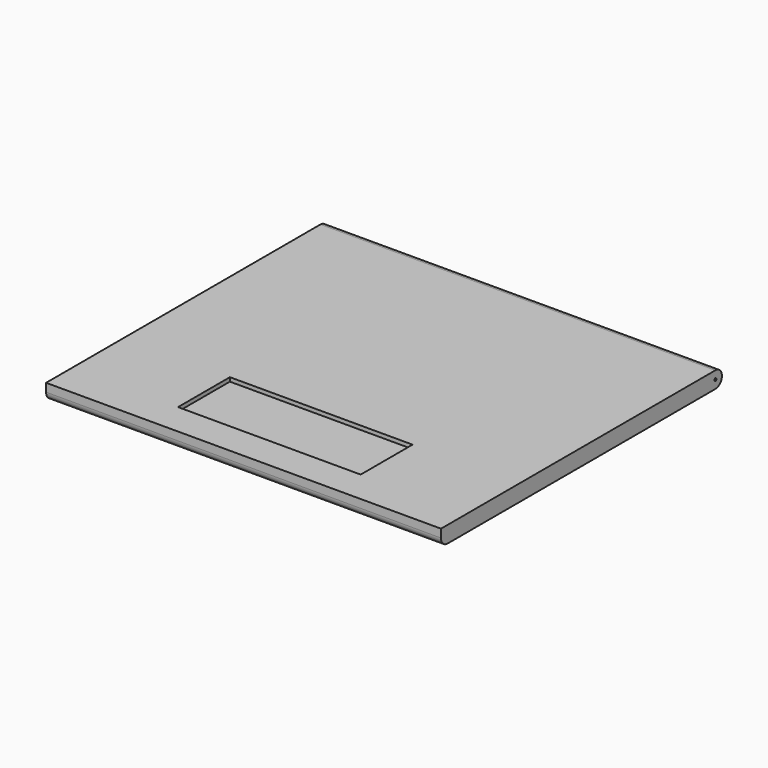
from build123d import *

# Parameters (mm, degrees)
F2_DEPTH = 5
F3_DEPTH = 1.2
F4_R     = 0.4
F5_DEPTH = 2.5
F6_R     = 0.4
F7_DEPTH = 5
F8_R     = 2.49999
F9_R     = 2.5


# Not quite as in the source:
# - a fillet or chamfer is up to 0.001 mm smaller than in the source, because OpenCascade refuses the exact size


with BuildPart() as f2:
    # F1 (on Top) → F2 (new body)
    with BuildSketch(Plane.XY):
        Polygon((-60, -46.1892857143), (-0.7, -46.1892857143), (60, -46.1892857143), (60, 60.5107142857), (0, 60.5107142857), (-60, 60.5107142857), align=None)
        Polygon((-27.75, -16.6892857143), (0, -16.6892857143), (27.75, -16.6892857143), (27.75, -36.3892857143), (-0.7, -36.3892857143), (-27.75, -36.3892857143), align=None, mode=Mode.SUBTRACT)
        Polygon((27.75, -16.6892857143), (0, -16.6892857143), (-27.75, -16.6892857143), (-27.75, -36.3892857143), (-0.7, -36.3892857143), (27.75, -36.3892857143), align=None)
    extrude(amount=-F2_DEPTH)

    # F1 (on Top) → F3 (cut)
    with BuildSketch(Plane.XY):
        Polygon((27.75, -16.6892857143), (0, -16.6892857143), (-27.75, -16.6892857143), (-27.75, -36.3892857143), (-0.7, -36.3892857143), (27.75, -36.3892857143), align=None)
    extrude(amount=-F3_DEPTH, mode=Mode.SUBTRACT)

    # F4 (on face) → F5 (cut, symmetric)
    with BuildSketch(Plane(origin=(-60, 0, 0), x_dir=(0, -1, 0), z_dir=(-1, 0, 0))):
        with Locations((-58.0107142857, -2.5)):
            Circle(F4_R)
    extrude(amount=F5_DEPTH, both=True, mode=Mode.SUBTRACT)

    # F6 (on face) → F7 (cut)
    with BuildSketch(Plane.YZ.offset(60)):
        with Locations((58.0107142857, -2.5)):
            Circle(F6_R)
    extrude(amount=-F7_DEPTH, mode=Mode.SUBTRACT)

    # F8 (radius 2.5 in the source; OpenCascade refuses exactly that, so slightly less here)
    f8_edges = [f2.edges().sort_by_distance(p)[0] for p in [
        (0, 60.510714, 0),
        (0, 60.510714, -5),
    ]]
    fillet(f8_edges, radius=F8_R)

    # F9
    f9_edges = [f2.edges().sort_by_distance(p)[0] for p in [
        (0, -46.189286, -5),
    ]]
    fillet(f9_edges, radius=F9_R)


solid = f2.part
